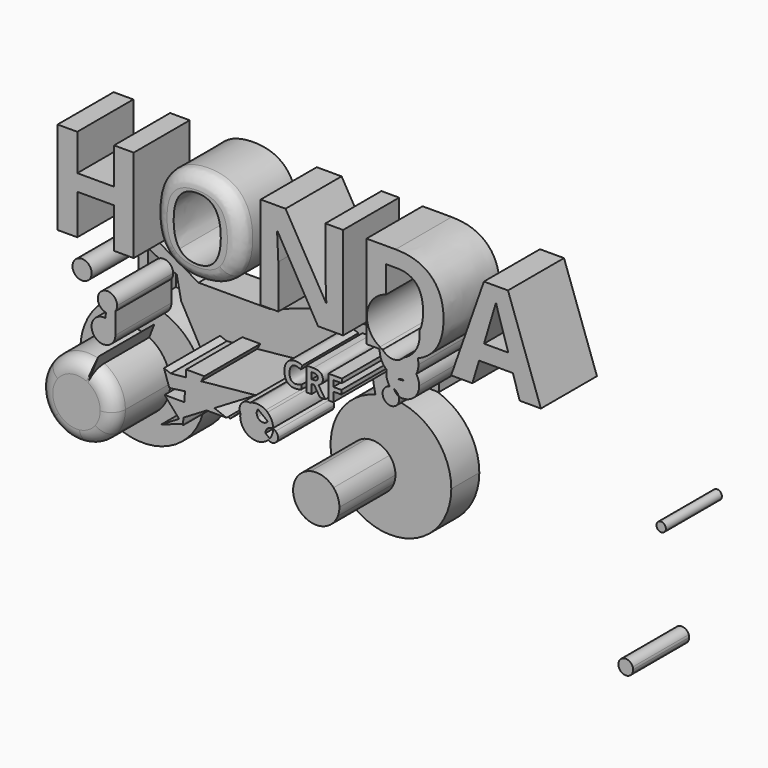
from build123d import *

# Parameters (mm, degrees)
F1_DEPTH     = 12.7
F2_R         = 3.4656393631
F2_R_2       = 1.7046990707
F2_TEXT_SIZE = 11.9919064067
F3_DEPTH     = 25.4
F4_R         = 5.08


# Not quite as in the source:
# - Text() gives the source's letters only with a copy of the font that has no kerning and outlines rounded to 1/6400 em; it was checked with that copy


with BuildPart() as f1:
    # F0 (on Front) → F1 (new body)
    with BuildSketch(Plane.XZ):
        Polygon((-7.7327229083, 0), (-33.6136706173, 0), (-41.5042005479, 0), (-39.926096797, -7.8905327246), (-22.2513023764, -39.7682860494), (14.6763911471, -6.6280472092), (28.8793519139, -6.6280472092), (38.0323678255, -6.6280472092), (53.4978099167, -6.6280472092), (53.4978099167, 6.3124261796), (10.8889359981, 6.3124261796), align=None)
        with BuildLine():
            Line((-33.6136706173, 0), (-49.1911599727, 8.9167358417))
            ThreePointArc((-49.1911599727, 8.9167358417), (-49.0836138425, 8.2496508856), (-49.0476290539, 7.5749112293))
            ThreePointArc((-49.0476290539, 7.5749112293), (-49.304530183, 5.7878698172), (-50.0544267833, 4.1455634245))
            Line((-50.0544267833, 4.1455634245), (-41.5042005479, 0))
            Line((-41.5042005479, 0), (-33.6136706173, 0))
        make_face()
        with BuildLine():
            ThreePointArc((-49.1911599727, 8.9167358417), (-60.3290284498, 11.5581748179), (-55.3915388882, 1.2310013949))
            ThreePointArc((-55.3915388882, 1.2310013949), (-53.5802220784, 1.4950820047), (-51.9197061658, 2.265337844))
            Line((-51.9197061658, 2.265337844), (-51.9197061658, 5.04994113))
            Line((-51.9197061658, 5.04994113), (-50.0544267833, 4.1455634245))
            ThreePointArc((-50.0544267833, 4.1455634245), (-49.304530183, 5.7878698172), (-49.0476290539, 7.5749112293))
            ThreePointArc((-49.0476290539, 7.5749112293), (-49.0836138425, 8.2496508856), (-49.1911599727, 8.9167358417))
        make_face()
        with BuildLine():
            Line((31.0644188899, -17.5534014317), (30.5209569773, -14.8360870582))
            ThreePointArc((30.5209569773, -14.8360870582), (22.8016029338, -53.3238912444), (58.0169072618, -35.9808281064))
            ThreePointArc((58.0169072618, -35.9808281064), (52.2645516652, -21.1952431781), (38.0323678255, -14.1846754595))
            Line((38.0323678255, -14.1846754595), (38.0323678255, -17.5534014317))
            Line((38.0323678255, -17.5534014317), (31.0644188899, -17.5534014317))
        make_face()
        with BuildLine():
            Line((38.0323678255, -6.6280472092), (28.8793519139, -6.6280472092))
            Line((28.8793519139, -6.6280472092), (30.5209569773, -14.8360870582))
            ThreePointArc((30.5209569773, -14.8360870582), (34.248390096, -14.1843740125), (38.0323678255, -14.1846754595))
            Line((38.0323678255, -14.1846754595), (38.0323678255, -6.6280472092))
        make_face()
        with BuildLine():
            ThreePointArc((38.0323678255, -14.1846754595), (34.248390096, -14.1843740125), (30.5209569773, -14.8360870582))
            Line((30.5209569773, -14.8360870582), (31.0644188899, -17.5534014317))
            Line((31.0644188899, -17.5534014317), (38.0323678255, -17.5534014317))
            Line((38.0323678255, -17.5534014317), (38.0323678255, -14.1846754595))
        make_face()
        with BuildLine():
            Line((-55.3915388882, 1.2310013949), (-55.3915388882, -12.4587648256))
            ThreePointArc((-55.3915388882, -12.4587648256), (-53.9717066576, -57.6637000926), (-51.9197061658, -12.4830472638))
            Line((-51.9197061658, -12.4830472638), (-51.9197061658, 2.265337844))
            ThreePointArc((-51.9197061658, 2.265337844), (-53.5802220784, 1.4950820047), (-55.3915388882, 1.2310013949))
        make_face()
    extrude(amount=-F1_DEPTH)

    # F2 (on Front) → F3 (join)
    with BuildSketch(Plane.XZ):
        with Locations((-55.5244684219, 7.3390468024)):
            Circle(F2_R)
        Polygon((-20.3333193984, -28.8411563333), (-26.7438944429, -32.6659530401), (-19.2087982655, -30.1156134303), align=None)
        with BuildLine():
            ThreePointArc((11.0659327715, -15.8007104203), (8.7972767618, -14.9049246061), (6.3596961465, -14.9911397987))
            Line((6.3596961465, -14.9911397987), (8.2503574618, -16.4433873123))
            ThreePointArc((8.2503574618, -16.4433873123), (9.5424129776, -15.615024952), (11.0659327715, -15.8007104203))
        make_face()
        with BuildLine():
            Line((8.2503574618, -16.4433873123), (6.3596961465, -14.9911397987))
            ThreePointArc((6.3596961465, -14.9911397987), (5.881282631, -15.1301590772), (5.4161247168, -15.3085798338))
            ThreePointArc((5.4161247168, -15.3085798338), (6.8824980035, -15.9750826456), (7.8525062628, -17.2609911146))
            ThreePointArc((7.8525062628, -17.2609911146), (8.0099772, -16.8320171117), (8.2503574618, -16.4433873123))
        make_face()
        Polygon((-20.3333193984, -28.8411563333), (-19.2087982655, -30.1156134303), (-18.9083775266, -30.0139325901), (-18.7716553459, -27.9094072337), align=None)
        Polygon((-18.9083775266, -30.0139325901), (-19.2087982655, -30.1156134303), (-18.9351327232, -30.425767666), align=None)
        Polygon((-25.5926717073, -22.8805579245), (-20.3333193984, -28.8411563333), (-18.7716553459, -27.9094072337), (-18.4449521098, -22.8805579245), align=None)
        Polygon((-18.4449521098, -22.8805579245), (-18.7716553459, -27.9094072337), (-10.3430202169, -22.8805579245), align=None)
        Polygon((-7.5691475634, -21.225558347), (-10.3430202169, -22.8805579245), (-3.1438225415, -22.8805579245), align=None)
        Polygon((-18.4449521098, -22.8805579245), (-10.3430202169, -22.8805579245), (-7.5691475634, -21.225558347), (-14.7648096943, -18.5344977519), (-14.9438586086, -18.8512764871), (-18.2128143814, -19.3073283819), align=None)
        Polygon((-14.7648096943, -18.5344977519), (-7.5691475634, -21.225558347), (4.8384941827, -13.8226799842), (7.5049912557, -12.2317448258), (-12.3231014672, -14.2145539698), align=None)
        Polygon((-18.0820115716, -17.2939182061), (-18.2128143814, -19.3073283819), (-14.9438586086, -18.8512764871), (-14.7648096943, -18.5344977519), align=None)
        Polygon((-23.8905889559, -20.0994344955), (-18.2128143814, -19.3073283819), (-18.0820115716, -17.2939182061), (-23.3637820538, -15.318621957), (-25.4384888951, -15.5260926277), align=None)
        Polygon((-18.0820115716, -17.2939182061), (-14.7648096943, -18.5344977519), (-12.3231014672, -14.2145539698), (-17.9183079055, -14.7740745774), align=None)
        Polygon((-23.3637820538, -15.318621957), (-18.0820115716, -17.2939182061), (-17.9183079055, -14.7740745774), align=None)
        Polygon((-17.9183079055, -14.7740745774), (-12.3231014672, -14.2145539698), (-11.2023828551, -12.2317448258), (-17.7531434104, -12.2317448258), align=None)
        Polygon((-25.8195598049, -14.4002010228), (-25.4384888951, -15.5260926277), (-23.3637820538, -15.318621957), align=None)
        with BuildLine():
            ThreePointArc((11.0659327715, -15.8007104203), (9.5424129776, -15.615024952), (8.2503574618, -16.4433873123))
            Line((8.2503574618, -16.4433873123), (11.8424194896, -19.2025082116))
            ThreePointArc((11.8424194896, -19.2025082116), (12.1907304547, -18.5514475317), (12.3110991498, -17.8229477619))
            ThreePointArc((12.3110991498, -17.8229477619), (12.1598720908, -17.0092515987), (11.7263874216, -16.3042252794))
            ThreePointArc((11.7263874216, -16.3042252794), (11.4049254743, -16.0409704046), (11.0659327715, -15.8007104203))
        make_face()
        with BuildLine():
            ThreePointArc((11.7263874216, -16.3042252794), (11.4194380858, -16.021934379), (11.0659327715, -15.8007104203))
            ThreePointArc((11.0659327715, -15.8007104203), (11.4049254743, -16.0409704046), (11.7263874216, -16.3042252794))
        make_face()
        with BuildLine():
            ThreePointArc((1.8790581004, -19.9134388255), (3.0501043864, -17.1520698912), (5.4161247168, -15.3085798338))
            ThreePointArc((5.4161247168, -15.3085798338), (2.2463076538, -16.5346606297), (1.8790581004, -19.9134388255))
        make_face()
        with BuildLine():
            ThreePointArc((7.8525062628, -17.2609911146), (6.8824980035, -15.9750826456), (5.4161247168, -15.3085798338))
            ThreePointArc((5.4161247168, -15.3085798338), (3.0501043864, -17.1520698912), (1.8790581004, -19.9134388255))
            ThreePointArc((1.8790581004, -19.9134388255), (4.4852977085, -21.7752477158), (7.4306807116, -20.5168613665))
            ThreePointArc((7.4306807116, -20.5168613665), (7.8591675927, -19.7745379308), (8.0799475068, -18.9463463346))
            ThreePointArc((8.0799475068, -18.9463463346), (7.8020226859, -18.1258283304), (7.8525062628, -17.2609911146))
        make_face()
        with BuildLine():
            ThreePointArc((12.3110991498, -17.8229477619), (12.1907304547, -18.5514475317), (11.8424194896, -19.2025082116))
            Line((11.8424194896, -19.2025082116), (13.7544967517, -20.6712056601))
            ThreePointArc((13.7544967517, -20.6712056601), (13.2001739357, -18.2742071937), (11.7263874216, -16.3042252794))
            ThreePointArc((11.7263874216, -16.3042252794), (12.1598720908, -17.0092515987), (12.3110991498, -17.8229477619))
        make_face()
        with BuildLine():
            Line((13.7544967517, -20.6712056601), (11.8424194896, -19.2025082116))
            ThreePointArc((11.8424194896, -19.2025082116), (9.8925554006, -20.0824277513), (8.0799475068, -18.9463463346))
            ThreePointArc((8.0799475068, -18.9463463346), (7.8591675927, -19.7745379308), (7.4306807116, -20.5168613665))
            Line((7.4306807116, -20.5168613665), (10.9644073575, -23.2311739162))
            ThreePointArc((10.9644073575, -23.2311739162), (11.8017352346, -21.4073746291), (13.7537170773, -20.9414039222))
            ThreePointArc((13.7537170773, -20.9414039222), (13.7551745863, -20.8652485493), (13.755660449, -20.78908078))
            ThreePointArc((13.755660449, -20.78908078), (13.7553695176, -20.730140348), (13.7544967517, -20.6712056601))
        make_face()
        with BuildLine():
            ThreePointArc((7.4306807116, -20.5168613665), (4.4852977085, -21.7752477158), (1.8790581004, -19.9134388255))
            ThreePointArc((1.8790581004, -19.9134388255), (5.0666176211, -26.1048876256), (11.9523159154, -25.064823714))
            ThreePointArc((11.9523159154, -25.064823714), (11.2380990725, -24.2666688426), (10.9644073575, -23.2311739162))
            Line((10.9644073575, -23.2311739162), (7.4306807116, -20.5168613665))
        make_face()
        with BuildLine():
            Line((14.652831676, -21.3612312346), (13.7544967517, -20.6712056601))
            ThreePointArc((13.7544967517, -20.6712056601), (13.7553695176, -20.730140348), (13.755660449, -20.78908078))
            ThreePointArc((13.755660449, -20.78908078), (13.7551745863, -20.8652485493), (13.7537170773, -20.9414039222))
            ThreePointArc((13.7537170773, -20.9414039222), (14.2262617553, -21.1020871278), (14.652831676, -21.3612312346))
        make_face()
        with BuildLine():
            ThreePointArc((10.9644073575, -23.2311739162), (11.2380990725, -24.2666688426), (11.9523159154, -25.064823714))
            ThreePointArc((11.9523159154, -25.064823714), (12.2476277526, -24.7556284042), (12.5200545516, -24.4260916688))
            Line((12.5200545516, -24.4260916688), (10.9644073575, -23.2311739162))
        make_face()
        with BuildLine():
            ThreePointArc((12.5200545516, -24.4260916688), (12.2476277526, -24.7556284042), (11.9523159154, -25.064823714))
            ThreePointArc((11.9523159154, -25.064823714), (12.8381463766, -25.4333611681), (13.797222002, -25.4071046293))
            Line((13.797222002, -25.4071046293), (12.5200545516, -24.4260916688))
        make_face()
        with BuildLine():
            ThreePointArc((15.5488486699, -23.1793116957), (15.3126796529, -22.1658691694), (14.652831676, -21.3612312346))
            ThreePointArc((14.652831676, -21.3612312346), (14.2262617553, -21.1020871278), (13.7537170773, -20.9414039222))
            ThreePointArc((13.7537170773, -20.9414039222), (13.4133645837, -22.7816278701), (12.5200545516, -24.4260916688))
            Line((12.5200545516, -24.4260916688), (13.797222002, -25.4071046293))
            ThreePointArc((13.797222002, -25.4071046293), (15.0585017297, -24.5962853492), (15.5488486699, -23.1793116957))
        make_face()
        with BuildLine():
            ThreePointArc((144.0968940704, -54.5208358441), (140.7111559708, -52.8474247407), (139.0377448675, -56.2331628404))
            Line((139.0377448675, -56.2331628404), (144.0968940704, -54.5208358441))
        make_face()
        with BuildLine():
            Line((144.0968940704, -54.5208358441), (139.0377448675, -56.2331628404))
            ThreePointArc((139.0377448675, -56.2331628404), (142.0011645185, -58.0120595072), (144.2378556698, -55.3769993422))
            ThreePointArc((144.2378556698, -55.3769993422), (144.2023796339, -54.9431542927), (144.0968940704, -54.5208358441))
        make_face()
        with BuildLine():
            ThreePointArc((56.1071860271, 6.2969433914), (54.4253769468, 1.0731827643), (59.4367492157, 3.3097660635))
            ThreePointArc((59.4367492157, 3.3097660635), (59.3974492098, 3.7941536842), (59.2805772139, 4.2658705422))
            ThreePointArc((59.2805772139, 4.2658705422), (57.5291300057, 5.0239955586), (56.1071860271, 6.2969433914))
        make_face()
        with BuildLine():
            ThreePointArc((56.1071860271, 6.2969433914), (57.5291300057, 5.0239955586), (59.2805772139, 4.2658705422))
            ThreePointArc((59.2805772139, 4.2658705422), (59.2761625355, 4.2789242932), (59.2716880386, 4.2919576611))
            ThreePointArc((59.2716880386, 4.2919576611), (58.2593677528, 5.0066356553), (57.6215328865, 6.0690497365))
            ThreePointArc((57.6215328865, 6.0690497365), (56.879121491, 6.2810898613), (56.1071860271, 6.2969433914))
        make_face()
        with BuildLine():
            ThreePointArc((59.2716880386, 4.2919576611), (59.2761625355, 4.2789242932), (59.2805772139, 4.2658705422))
            ThreePointArc((59.2805772139, 4.2658705422), (59.3510578372, 4.2485042768), (59.4217447752, 4.2319978469))
            ThreePointArc((59.4217447752, 4.2319978469), (59.3463132652, 4.2609688428), (59.2716880386, 4.2919576611))
        make_face()
        with BuildLine():
            ThreePointArc((54.9158672093, 11.2965345115), (54.9448027467, 8.6616981459), (56.1071860271, 6.2969433914))
            ThreePointArc((56.1071860271, 6.2969433914), (56.879121491, 6.2810898613), (57.6215328865, 6.0690497365))
            ThreePointArc((57.6215328865, 6.0690497365), (57.6596067986, 8.1372838388), (59.0254851788, 9.6908018385))
            ThreePointArc((59.0254851788, 9.6908018385), (56.8414989893, 10.163059618), (54.9158672093, 11.2965345115))
        make_face()
        with BuildLine():
            ThreePointArc((57.6215328865, 6.0690497365), (58.6338531525, 5.3543717239), (59.2716880386, 4.2919576611))
            ThreePointArc((59.2716880386, 4.2919576611), (59.3463132652, 4.2609688428), (59.4217447752, 4.2319978469))
            ThreePointArc((59.4217447752, 4.2319978469), (60.1858173934, 4.1099907527), (60.9592576445, 4.0880163335))
            ThreePointArc((60.9592576445, 4.0880163335), (62.7552783216, 5.1105821282), (63.4660340885, 7.0512411185))
            ThreePointArc((63.4660340885, 7.0512411185), (62.8613094451, 8.8591234536), (61.2905421888, 9.9393181855))
            ThreePointArc((61.2905421888, 9.9393181855), (60.1681450932, 9.7227191251), (59.0254851788, 9.6908018385))
            ThreePointArc((59.0254851788, 9.6908018385), (57.6596067986, 8.1372838388), (57.6215328865, 6.0690497365))
        make_face()
        with BuildLine():
            ThreePointArc((60.9592576445, 4.0880163335), (60.1858173934, 4.1099907527), (59.4217447752, 4.2319978469))
            ThreePointArc((59.4217447752, 4.2319978469), (60.1810937555, 4.0595491788), (60.9592576445, 4.0880163335))
        make_face()
        with BuildLine():
            ThreePointArc((52.3799228636, 17.1244423836), (52.9520293994, 13.9076908457), (54.9158672093, 11.2965345115))
            ThreePointArc((54.9158672093, 11.2965345115), (56.2977177627, 14.0130804753), (58.8420527676, 15.6910233552))
            ThreePointArc((58.8420527676, 15.6910233552), (56.0114015567, 15.6108890227), (53.6180432442, 17.1244423836))
            Line((53.6180432442, 17.1244423836), (52.3799228636, 17.1244423836))
        make_face()
        with BuildLine():
            ThreePointArc((58.8420527676, 15.6910233552), (56.2977177627, 14.0130804753), (54.9158672093, 11.2965345115))
            ThreePointArc((54.9158672093, 11.2965345115), (56.8414989893, 10.163059618), (59.0254851788, 9.6908018385))
            ThreePointArc((59.0254851788, 9.6908018385), (60.1335424874, 10.0380982779), (61.2905421888, 9.9393181855))
            ThreePointArc((61.2905421888, 9.9393181855), (63.82373091, 11.245327823), (65.6306764112, 13.4493364949))
            ThreePointArc((65.6306764112, 13.4493364949), (62.6098801732, 15.7013177162), (58.8420527676, 15.6910233552))
        make_face()
        with BuildLine():
            ThreePointArc((63.4660340885, 7.0512411185), (62.7552783216, 5.1105821282), (60.9592576445, 4.0880163335))
            ThreePointArc((60.9592576445, 4.0880163335), (65.0313194245, 5.9070915445), (66.7003121561, 10.0429330581))
            ThreePointArc((66.7003121561, 10.0429330581), (66.4266177804, 11.828129476), (65.6306764112, 13.4493364949))
            ThreePointArc((65.6306764112, 13.4493364949), (63.82373091, 11.245327823), (61.2905421888, 9.9393181855))
            ThreePointArc((61.2905421888, 9.9393181855), (62.8613094451, 8.8591234536), (63.4660340885, 7.0512411185))
        make_face()
        with BuildLine():
            ThreePointArc((61.0876135348, 17.2629962453), (60.0781406733, 16.3151501855), (58.8420527676, 15.6910233552))
            ThreePointArc((58.8420527676, 15.6910233552), (62.6098801732, 15.7013177162), (65.6306764112, 13.4493364949))
            ThreePointArc((65.6306764112, 13.4493364949), (66.2303982017, 15.0329071777), (66.4342442576, 16.7139214901))
            ThreePointArc((66.4342442576, 16.7139214901), (66.3661851402, 17.6899895067), (66.1633249899, 18.6471669072))
            add(Edge.make_bspline(
                [(66.1633249899, 18.6471669072), (64.0211964645, 17.7879612829), (61.4189010583, 17.4135671221)],
                knots=[0.413185892, 0.413185892, 0.413185892, 0.7442989556, 0.7442989556, 0.7442989556], degree=2))
            ThreePointArc((61.4189010583, 17.4135671221), (61.2539732609, 17.3367064119), (61.0876135348, 17.2629962453))
        make_face()
        with BuildLine():
            Line((47.5884310771, 17.1244423836), (52.3799228636, 17.1244423836))
            ThreePointArc((52.3799228636, 17.1244423836), (52.4077359551, 17.4611259151), (52.4516845408, 17.7960854503))
            ThreePointArc((52.4516845408, 17.7960854503), (47.8086422031, 27.2838164806), (54.7299859229, 35.2631575165))
            Line((54.7299859229, 35.2631575165), (54.7299859229, 44.9462891771))
            Line((54.7299859229, 44.9462891771), (58.5255491278, 44.9462891771))
            add(Edge.make_bspline(
                [(68.1065824606, 34.097611434), (68.1065824606, 44.9462891771), (58.5255491278, 44.9462891771)],
                knots=[0, 0, 0, 1, 1, 1], degree=2))
            add(Edge.make_bspline(
                [(66.7485997068, 27.518269432), (68.1065824606, 30.0789946905), (68.1065824606, 34.097611434)],
                knots=[0.6372155948, 0.6372155948, 0.6372155948, 1, 1, 1], degree=2))
            ThreePointArc((66.7485997068, 27.518269432), (66.8339791577, 26.7845455173), (66.8624956403, 26.0464213789))
            ThreePointArc((66.8624956403, 26.0464213789), (66.4407009491, 23.2370089097), (65.2125090542, 20.6753192617))
            ThreePointArc((65.2125090542, 20.6753192617), (65.7691779525, 19.6993389343), (66.1633249899, 18.6471669072))
            add(Edge.make_bspline(
                [(70.7929568066, 21.546457768), (68.8364218344, 19.719343397), (66.1633249899, 18.6471669072)],
                knots=[0, 0, 0, 0.413185892, 0.413185892, 0.413185892], degree=2))
            add(Edge.make_bspline(
                [(75.5281982808, 34.2818620751), (75.5281982808, 25.9684731524), (70.7929568066, 21.546457768)],
                knots=[0, 0, 0, 1, 1, 1], degree=2))
            add(Edge.make_bspline(
                [(70.9661524092, 46.4460893949), (75.5281982808, 42.0940892541), (75.5281982808, 34.2818620751)],
                knots=[0, 0, 0, 1, 1, 1], degree=2))
            add(Edge.make_bspline(
                [(58.1570478458, 50.7980895357), (66.4041065376, 50.7980895357), (70.9661524092, 46.4460893949)],
                knots=[0, 0, 0, 1, 1, 1], degree=2))
            Line((58.1570478458, 50.7980895357), (47.5884310771, 50.7980895357))
            Line((47.5884310771, 50.7980895357), (47.5884310771, 17.1244423836))
        make_face()
        with BuildLine():
            ThreePointArc((52.4516845408, 17.7960854503), (52.4077359551, 17.4611259151), (52.3799228636, 17.1244423836))
            Line((52.3799228636, 17.1244423836), (53.6180432442, 17.1244423836))
            ThreePointArc((53.6180432442, 17.1244423836), (53.5599618708, 17.19318664), (53.5031654121, 17.2629962453))
            ThreePointArc((53.5031654121, 17.2629962453), (52.9692060027, 17.5133295016), (52.4516845408, 17.7960854503))
        make_face()
        with BuildLine():
            ThreePointArc((65.2125090542, 20.6753192617), (63.5326930953, 18.7920734456), (61.4189010583, 17.4135671221))
            add(Edge.make_bspline(
                [(66.1633249899, 18.6471669072), (64.0211964645, 17.7879612829), (61.4189010583, 17.4135671221)],
                knots=[0.413185892, 0.413185892, 0.413185892, 0.7442989556, 0.7442989556, 0.7442989556], degree=2))
            ThreePointArc((66.1633249899, 18.6471669072), (65.7691779525, 19.6993389343), (65.2125090542, 20.6753192617))
        make_face()
        with BuildLine():
            ThreePointArc((-46.69328711, -43.8748629365), (-44.5899165618, -39.9432558479), (-43.8630374405, -35.5440117419))
            ThreePointArc((-43.8630374405, -35.5440117419), (-43.891178, -34.6671350523), (-43.9754838718, -33.7938669722))
            Line((-43.9754838718, -33.7938669722), (-57.5391091406, -35.5440117419))
            Line((-57.5391091406, -35.5440117419), (-46.69328711, -43.8748629365))
        make_face()
        with BuildLine():
            ThreePointArc((-47.1164325225, -5.3717028782), (-52.0544769687, -9.2664310453), (-47.8651528718, -13.9571403796))
            ThreePointArc((-47.8651528718, -13.9571403796), (-44.7407302825, -12.7332822113), (-43.436627835, -9.6414927393))
            ThreePointArc((-43.436627835, -9.6414927393), (-44.4835127816, -6.823156883), (-47.1164325225, -5.3717028782))
        make_face()
        with BuildLine():
            Line((-57.5391091406, -35.5440117419), (-43.9754838718, -33.7938669722))
            ThreePointArc((-43.9754838718, -33.7938669722), (-46.4128866606, -27.5915209075), (-51.4921266975, -23.2774335523))
            ThreePointArc((-51.4921266975, -23.2774335523), (-51.6383553996, -23.2064251693), (-51.7854177831, -23.1371598886))
            Line((-51.7854177831, -23.1371598886), (-57.5391091406, -35.5440117419))
        make_face()
        with BuildLine():
            ThreePointArc((-55.7889643709, -49.1076370107), (-50.7192795213, -47.3983299893), (-46.69328711, -43.8748629365))
            Line((-46.69328711, -43.8748629365), (-57.5391091406, -35.5440117419))
            Line((-57.5391091406, -35.5440117419), (-55.7889643709, -49.1076370107))
        make_face()
        with BuildLine():
            ThreePointArc((-51.7854177831, -23.1371598886), (-51.6383553996, -23.2064251693), (-51.4921266975, -23.2774335523))
            Line((-51.4921266975, -23.2774335523), (-49.6229203613, -18.4741038645))
            Line((-49.6229203613, -18.4741038645), (-51.7854177831, -23.1371598886))
        make_face()
        with BuildLine():
            Line((-68.3849311713, -27.2131605473), (-57.5391091406, -35.5440117419))
            Line((-57.5391091406, -35.5440117419), (-51.7854177831, -23.1371598886))
            ThreePointArc((-51.7854177831, -23.1371598886), (-60.8003809846, -22.2624815926), (-68.3849311713, -27.2131605473))
        make_face()
        with BuildLine():
            Line((-67.7713799412, -44.6179067937), (-57.5391091406, -35.5440117419))
            Line((-57.5391091406, -35.5440117419), (-68.3849311713, -27.2131605473))
            ThreePointArc((-68.3849311713, -27.2131605473), (-71.206691126, -36.0258206474), (-67.7713799412, -44.6179067937))
        make_face()
        with BuildLine():
            Line((-55.7889643709, -49.1076370107), (-57.5391091406, -35.5440117419))
            Line((-57.5391091406, -35.5440117419), (-67.7713799412, -44.6179067937))
            ThreePointArc((-67.7713799412, -44.6179067937), (-62.3376542176, -48.3506077881), (-55.7889643709, -49.1076370107))
        make_face()
        with BuildLine():
            Line((-46.8319804795, -3.465872496), (-47.1164325225, -5.3717028782))
            ThreePointArc((-47.1164325225, -5.3717028782), (-44.4835127816, -6.823156883), (-43.436627835, -9.6414927393))
            Line((-43.436627835, -9.6414927393), (-43.436627835, -1.9991606467))
            ThreePointArc((-43.436627835, -1.9991606467), (-44.9250414475, -3.2169475762), (-46.8319804795, -3.465872496))
        make_face()
        with BuildLine():
            ThreePointArc((-42.8104226794, 0), (-48.6023852402, 2.6544867347), (-46.8319804795, -3.465872496))
            ThreePointArc((-46.8319804795, -3.465872496), (-44.9250414475, -3.2169475762), (-43.436627835, -1.9991606467))
            ThreePointArc((-43.436627835, -1.9991606467), (-42.9706364273, -1.0474703084), (-42.8104226794, 0))
        make_face()
        with BuildLine():
            ThreePointArc((37.2375028695, -41.0735036689), (37.6351582852, -39.627729059), (37.7691362444, -38.1342619658))
            ThreePointArc((37.7691362444, -38.1342619658), (37.2213919528, -35.1522957459), (35.6496707023, -32.5596448523))
            Line((35.6496707023, -32.5596448523), (29.3782260269, -38.1342619658))
            Line((29.3782260269, -38.1342619658), (37.2375028695, -41.0735036689))
        make_face()
        with BuildLine():
            Line((29.3782260269, -38.1342619658), (35.6496707023, -32.5596448523))
            ThreePointArc((35.6496707023, -32.5596448523), (31.894524898, -30.129537469), (27.42436253, -29.9740051246))
            Line((27.42436253, -29.9740051246), (29.3782260269, -38.1342619658))
        make_face()
        with BuildLine():
            ThreePointArc((29.3782260269, -46.5251721832), (34.1607181094, -45.0288354666), (37.2375028695, -41.0735036689))
            Line((37.2375028695, -41.0735036689), (29.3782260269, -38.1342619658))
            Line((29.3782260269, -38.1342619658), (29.3782260269, -46.5251721832))
        make_face()
        with BuildLine():
            Line((29.3782260269, -38.1342619658), (27.42436253, -29.9740051246))
            ThreePointArc((27.42436253, -29.9740051246), (23.3063417157, -32.3429240211), (21.1347314033, -36.5683211405))
            Line((21.1347314033, -36.5683211405), (29.3782260269, -38.1342619658))
        make_face()
        with BuildLine():
            Line((29.3782260269, -46.5251721832), (29.3782260269, -38.1342619658))
            Line((29.3782260269, -38.1342619658), (21.1347314033, -36.5683211405))
            ThreePointArc((21.1347314033, -36.5683211405), (22.9149821375, -43.4853228609), (29.3782260269, -46.5251721832))
        make_face()
        with Locations((154.4199585915, -6.4756297506)):
            Circle(F2_R_2)
        with Locations((17.1366091818, -5.3244065493)):
            Text('CRF', F2_TEXT_SIZE, font='Open Sans', font_style=FontStyle.BOLD, text_align=(TextAlign.LEFT, TextAlign.BOTTOM))
        Polygon((-43.9178072771, 17.1244423836), (-36.7983625082, 17.1244423836), (-36.7983625082, 50.7980895357), (-43.9178072771, 50.7980895357), (-43.9178072771, 37.5983736133), (-57.250183661, 37.5983736133), (-57.250183661, 50.7980895357), (-64.3917385068, 50.7980895357), (-64.3917385068, 17.1244423836), (-57.250183661, 17.1244423836), (-57.250183661, 31.658132947), (-43.9178072771, 31.658132947), align=None)
        with BuildLine():
            add(Edge.make_bspline(
                [(2.2627733872, 34.0091711263), (2.2627733872, 25.6441920242), (-1.8828660357, 21.1521613963)],
                knots=[0, 0, 0, 1, 1, 1], degree=2))
            add(Edge.make_bspline(
                [(-1.8497009203, 46.8588108308), (2.2627733872, 42.3888902798), (2.2627733872, 34.0091711263)],
                knots=[0, 0, 0, 1, 1, 1], degree=2))
            add(Edge.make_bspline(
                [(-13.7228122274, 51.3287313818), (-5.9621752278, 51.3287313818), (-1.8497009203, 46.8588108308)],
                knots=[0, 0, 0, 1, 1, 1], degree=2))
            add(Edge.make_bspline(
                [(-25.6401436883, 46.895660959), (-21.483449227, 51.3287313818), (-13.7228122274, 51.3287313818)],
                knots=[0, 0, 0, 1, 1, 1], degree=2))
            add(Edge.make_bspline(
                [(-29.7968381496, 34.0533912802), (-29.7968381496, 42.4625905362), (-25.6401436883, 46.895660959)],
                knots=[0, 0, 0, 1, 1, 1], degree=2))
            add(Edge.make_bspline(
                [(-25.6511987267, 21.1521613963), (-29.7968381496, 25.6441920242), (-29.7968381496, 34.0533912802)],
                knots=[0, 0, 0, 1, 1, 1], degree=2))
            add(Edge.make_bspline(
                [(-13.7670323812, 16.6601307683), (-21.5055593039, 16.6601307683), (-25.6511987267, 21.1521613963)],
                knots=[0, 0, 0, 1, 1, 1], degree=2))
            add(Edge.make_bspline(
                [(-1.8828660357, 21.1521613963), (-6.0285054585, 16.6601307683), (-13.7670323812, 16.6601307683)],
                knots=[0, 0, 0, 1, 1, 1], degree=2))
        make_face()
        with BuildLine():
            add(Edge.make_bspline(
                [(-22.3088920987, 34.0091711263), (-22.3088920987, 28.3637314856), (-20.1678996501, 25.5078465499)],
                knots=[0, 0, 0, 1, 1, 1], degree=2))
            add(Edge.make_bspline(
                [(-20.1457895732, 42.5141807156), (-22.3088920987, 39.6472407414), (-22.3088920987, 34.0091711263)],
                knots=[0, 0, 0, 1, 1, 1], degree=2))
            add(Edge.make_bspline(
                [(-13.7228122274, 45.3811206899), (-17.9826870477, 45.3811206899), (-20.1457895732, 42.5141807156)],
                knots=[0, 0, 0, 1, 1, 1], degree=2))
            add(Edge.make_bspline(
                [(-5.2251726637, 34.0091711263), (-5.2251726637, 45.3811206899), (-13.7228122274, 45.3811206899)],
                knots=[0, 0, 0, 1, 1, 1], degree=2))
            add(Edge.make_bspline(
                [(-13.7670323812, 22.6519616141), (-5.2251726637, 22.6519616141), (-5.2251726637, 34.0091711263)],
                knots=[0, 0, 0, 1, 1, 1], degree=2))
            add(Edge.make_bspline(
                [(-20.1678996501, 25.5078465499), (-18.0269072015, 22.6519616141), (-13.7670323812, 22.6519616141)],
                knots=[0, 0, 0, 1, 1, 1], degree=2))
        make_face(mode=Mode.SUBTRACT)
        with BuildLine():
            Line((30.0404000267, 17.1244423836), (39.1129015904, 17.1244423836))
            Line((39.1129015904, 17.1244423836), (39.1129015904, 50.7980895357))
            Line((39.1129015904, 50.7980895357), (32.6862392317, 50.7980895357))
            Line((32.6862392317, 50.7980895357), (32.6862392317, 34.856724075))
            add(Edge.make_bspline(
                [(33.0326304368, 25.5778617935), (32.6862392317, 32.1445546393), (32.6862392317, 34.856724075)],
                knots=[0, 0, 0, 1, 1, 1], degree=2))
            Line((33.0326304368, 25.5778617935), (32.8704898727, 25.5778617935))
            Line((32.8704898727, 25.5778617935), (18.2483590017, 50.7980895357))
            Line((18.2483590017, 50.7980895357), (9.2421876689, 50.7980895357))
            Line((9.2421876689, 50.7980895357), (9.2421876689, 17.1244423836))
            Line((9.2421876689, 17.1244423836), (15.6246298737, 17.1244423836))
            Line((15.6246298737, 17.1244423836), (15.6246298737, 32.969997511))
            add(Edge.make_bspline(
                [(15.1824283352, 42.5952509977), (15.6246298737, 35.8516775365), (15.6246298737, 32.969997511)],
                knots=[0, 0, 0, 1, 1, 1], degree=2))
            Line((15.1824283352, 42.5952509977), (15.3887890532, 42.5952509977))
            Line((15.3887890532, 42.5952509977), (30.0404000267, 17.1244423836))
        make_face()
        Polygon((100.6820957923, 25.1430302807), (103.1215742793, 17.1244423836), (110.8158810481, 17.1244423836), (98.8838095359, 50.9381200229), (90.1576991774, 50.9381200229), (78.2698478191, 17.1244423836), (85.9641545879, 17.1244423836), (88.403633075, 25.1430302807), align=None)
        with BuildLine():
            add(Edge.make_bspline(
                [(98.9722498436, 31.1274911009), (95.5894080746, 42.0203889977), (95.1619465874, 43.450173972)],
                knots=[0, 0, 0, 1, 1, 1], degree=2))
            Line((98.9722498436, 31.1274911009), (90.2019193313, 31.1274911009))
            add(Edge.make_bspline(
                [(94.5502344592, 45.705401818), (93.7911218183, 42.7573915618), (90.2019193313, 31.1274911009)],
                knots=[0, 0, 0, 1, 1, 1], degree=2))
            add(Edge.make_bspline(
                [(95.1619465874, 43.450173972), (94.7344851003, 44.8799589463), (94.5502344592, 45.705401818)],
                knots=[0, 0, 0, 1, 1, 1], degree=2))
        make_face(mode=Mode.SUBTRACT)
    extrude(amount=F3_DEPTH)

    # F4
    f4_edges = [f1.edges().sort_by_distance(p)[0] for p in [
        (-29.796813, -25.4, 34.012138),
        (-63.439863, -25.4, -47.881598),
    ]]
    fillet(f4_edges, radius=F4_R)


solid = f1.part
